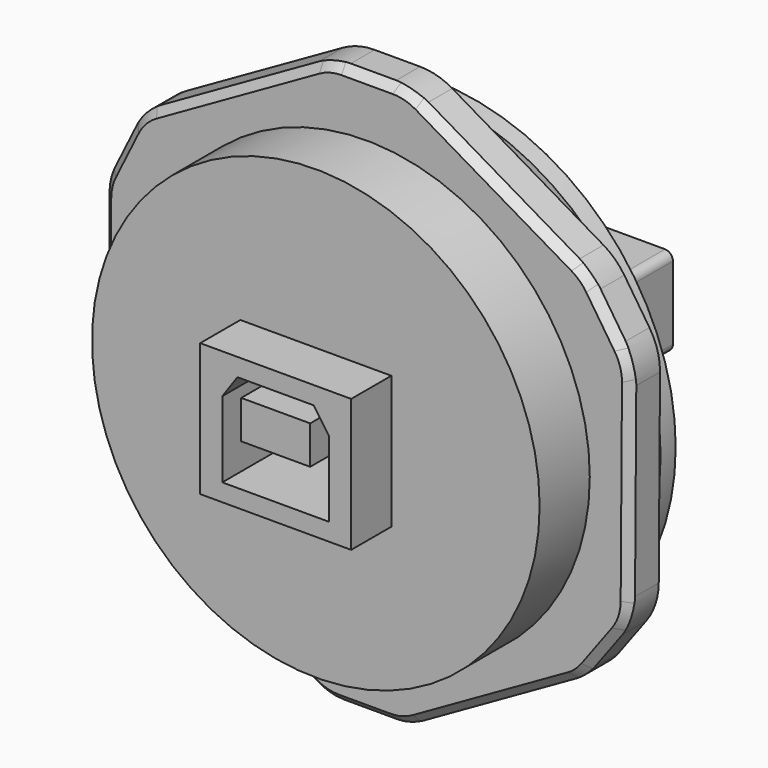
from build123d import *

# Parameters (mm, degrees)
F0_R      = 17.85
F1_DEPTH  = 5
F4_DEPTH  = 3
F5_SIZE   = 0.635
F6_F1_R   = 5.08
F6_F2_R   = 5.08
F6_F3_R   = 5.08
F6_F4_R   = 5.08
F6_F5_R   = 5.08
F6_F6_R   = 5.08
F6_F7_R   = 5.08
F6_F8_R   = 5.08
F6_F9_R   = 5.08
F6_F10_R  = 5.08
F6_F11_R  = 5.08
F6_F12_R  = 5.08
F6_F13_R  = 5.08
F6_F14_R  = 5.08
F6_F15_R  = 5.08
F6_F16_R  = 5.08
F6_F17_R  = 5.08
F6_F18_R  = 5.08
F6_F19_R  = 5.08
F6_F20_R  = 5.08
F6_F21_R  = 5.08
F6_F22_R  = 5.08
F6_F23_R  = 5.08
F6_F24_R  = 5.08
F7_R      = 19.5
F8_DEPTH  = 1.5
F9_W      = 12.04
F9_H      = 10.6
F9_W_2    = 5.5
F9_H_2    = 3.05
F10_DEPTH = 4
F11_DEPTH = 3
F12_W     = 10
F12_H     = 1.5
F13_DEPTH = 15.1


with BuildPart() as f1:
    # F0 (on Front) → F1 (new body, symmetric)
    with BuildSketch(Plane.XZ):
        Circle(F0_R)
    extrude(amount=F1_DEPTH, both=True)

    # F3 (on offset) → F4 (join)
    with BuildSketch(Plane(origin=(0, 3, 0), x_dir=(-1, 0, 0), z_dir=(0, 1, 0))):
        Polygon((-3.2903481497, 22.4154013943), (-17.5555016387, 14.0492031865), (-21.0601798177, 8.7539476816), (-20.9370838593, -9.2984309735), (-17.1594677511, -14.4025583758), (-3.0596518503, -22.4154013943), (3.2903481497, -22.4154013943), (18.0473649217, -13.7607362086), (21.0561899697, -8.1688249226), (20.9448872454, 8.1540418144), (18.1346734923, 13.8483546493), (3.0596518503, 22.4154013943), align=None)
    extrude(amount=-F4_DEPTH)

    # F5
    f5_edges = [f1.edges().sort_by_distance(p)[0] for p in [
        (10.422925, 0, 18.232302),
        (19.307841, 0, 11.401575),
        (20.998632, 0, -0.272242),
        (19.048276, 0, -11.850495),
        (10.10956, 0, -18.40898),
        (-0.115348, 0, -22.415401),
        (-10.668857, 0, -18.088069),
        (-19.551777, 0, -10.964781),
        (-21.000539, 0, -0.007392),
        (-19.53978, 0, 11.001198),
        (-10.597163, 0, 18.131878),
        (0.115348, 0, 22.415401),
    ]]
    chamfer(f5_edges, length=F5_SIZE)

    # F6: fillet of radius 5.08 on 24 edges, made by hand

    # F6_f1
    f6_f1_edges = [f1.edges().sort_by_distance(p)[0] for p in [
        (-20.9448872454, 1.8175, 8.1540418144),
    ]]
    fillet(f6_f1_edges, radius=F6_F1_R)

    # F6_f2
    f6_f2_edges = [f1.edges().sort_by_distance(p)[0] for p in [
        (-18.1346734923, 1.8175, 13.8483546493),
    ]]
    fillet(f6_f2_edges, radius=F6_F2_R)

    # F6_f3
    f6_f3_edges = [f1.edges().sort_by_distance(p)[0] for p in [
        (-21.0561899697, 1.8175, -8.1688249226),
    ]]
    fillet(f6_f3_edges, radius=F6_F3_R)

    # F6_f4
    f6_f4_edges = [f1.edges().sort_by_distance(p)[0] for p in [
        (-20.5635101748, 0.2530156874, 8.0636856851),
    ]]
    fillet(f6_f4_edges, radius=F6_F4_R)

    # F6_f5
    f6_f5_edges = [f1.edges().sort_by_distance(p)[0] for p in [
        (-17.80801976, 0.205710524, 13.540221636),
    ]]
    fillet(f6_f5_edges, radius=F6_F5_R)

    # F6_f6
    f6_f6_edges = [f1.edges().sort_by_distance(p)[0] for p in [
        (-3.0596518503, 1.8175, 22.4154013943),
    ]]
    fillet(f6_f6_edges, radius=F6_F6_R)

    # F6_f7
    f6_f7_edges = [f1.edges().sort_by_distance(p)[0] for p in [
        (-18.0473649217, 1.8175, -13.7607362086),
    ]]
    fillet(f6_f7_edges, radius=F6_F7_R)

    # F6_f8
    f6_f8_edges = [f1.edges().sort_by_distance(p)[0] for p in [
        (-20.6589027008, 0.2383946915, -8.0701656315),
    ]]
    fillet(f6_f8_edges, radius=F6_F8_R)

    # F6_f9
    f6_f9_edges = [f1.edges().sort_by_distance(p)[0] for p in [
        (-2.9534511203, 0.2331786487, 22.013580043),
    ]]
    fillet(f6_f9_edges, radius=F6_F9_R)

    # F6_f10
    f6_f10_edges = [f1.edges().sort_by_distance(p)[0] for p in [
        (3.2903481497, 1.8175, 22.4154013943),
    ]]
    fillet(f6_f10_edges, radius=F6_F10_R)

    # F6_f11
    f6_f11_edges = [f1.edges().sort_by_distance(p)[0] for p in [
        (-3.2903481497, 1.8175, -22.4154013943),
    ]]
    fillet(f6_f11_edges, radius=F6_F11_R)

    # F6_f12
    f6_f12_edges = [f1.edges().sort_by_distance(p)[0] for p in [
        (17.5555016387, 1.8175, 14.0492031865),
    ]]
    fillet(f6_f12_edges, radius=F6_F12_R)

    # F6_f13
    f6_f13_edges = [f1.edges().sort_by_distance(p)[0] for p in [
        (3.0596518503, 1.8175, -22.4154013943),
    ]]
    fillet(f6_f13_edges, radius=F6_F13_R)

    # F6_f14
    f6_f14_edges = [f1.edges().sort_by_distance(p)[0] for p in [
        (21.0601798177, 1.8175, 8.7539476816),
    ]]
    fillet(f6_f14_edges, radius=F6_F14_R)

    # F6_f15
    f6_f15_edges = [f1.edges().sort_by_distance(p)[0] for p in [
        (17.1594677511, 1.8175, -14.4025583758),
    ]]
    fillet(f6_f15_edges, radius=F6_F15_R)

    # F6_f16
    f6_f16_edges = [f1.edges().sort_by_distance(p)[0] for p in [
        (20.9370838593, 1.8175, -9.2984309735),
    ]]
    fillet(f6_f16_edges, radius=F6_F16_R)

    # F6_f17
    f6_f17_edges = [f1.edges().sort_by_distance(p)[0] for p in [
        (-17.7394232188, 0.2231799565, -13.4639178232),
    ]]
    fillet(f6_f17_edges, radius=F6_F17_R)

    # F6_f18
    f6_f18_edges = [f1.edges().sort_by_distance(p)[0] for p in [
        (3.1799932747, 0.2286960306, 22.009097425),
    ]]
    fillet(f6_f18_edges, radius=F6_F18_R)

    # F6_f19
    f6_f19_edges = [f1.edges().sort_by_distance(p)[0] for p in [
        (17.2850276, 0.2518471741, 13.7636444987),
    ]]
    fillet(f6_f19_edges, radius=F6_F19_R)

    # F6_f20
    f6_f20_edges = [f1.edges().sort_by_distance(p)[0] for p in [
        (20.6315309968, 0.2072299177, 8.6265365553),
    ]]
    fillet(f6_f20_edges, radius=F6_F20_R)

    # F6_f21
    f6_f21_edges = [f1.edges().sort_by_distance(p)[0] for p in [
        (20.4954738766, 0.1923957856, -9.1511150124),
    ]]
    fillet(f6_f21_edges, radius=F6_F21_R)

    # F6_f22
    f6_f22_edges = [f1.edges().sort_by_distance(p)[0] for p in [
        (16.9069384559, 0.262522864, -14.1176463871),
    ]]
    fillet(f6_f22_edges, radius=F6_F22_R)

    # F6_f23
    f6_f23_edges = [f1.edges().sort_by_distance(p)[0] for p in [
        (2.9534511203, 0.2331786487, -22.013580043),
    ]]
    fillet(f6_f23_edges, radius=F6_F23_R)

    # F6_f24
    f6_f24_edges = [f1.edges().sort_by_distance(p)[0] for p in [
        (-3.1799932747, 0.2286960306, -22.009097425),
    ]]
    fillet(f6_f24_edges, radius=F6_F24_R)

    # F7 (on face) → F8 (join)
    with BuildSketch(Plane(origin=(0, 5, 0), x_dir=(-1, 0, 0), z_dir=(0, 1, 0))):
        Circle(F7_R)
    extrude(amount=F8_DEPTH)

    # F9 (on face) → F10 (join)
    with BuildSketch(Plane.XZ.offset(5)):
        Rectangle(F9_W, F9_H)
        Polygon((4.2387, -3.903), (-4.2613, -3.903), (-4.2613, 2.1469455678), (-3.0499028451, 3.877), (3.0273028451, 3.877), (4.2387, 2.1469455678), align=None, mode=Mode.SUBTRACT)
        with Locations((0, 0.9936958086)):
            Rectangle(F9_W_2, F9_H_2)
    extrude(amount=F10_DEPTH)

    # F9 (on face) → F11 (cut)
    with BuildSketch(Plane.XZ.offset(5)):
        Polygon((-4.2613, 2.1469455678), (-4.2613, -3.903), (4.2387, -3.903), (4.2387, 2.1469455678), (3.0273028451, 3.877), (-3.0499028451, 3.877), align=None)
        with Locations((0, 0.9936958086)):
            Rectangle(F9_W_2, F9_H_2, mode=Mode.SUBTRACT)
    extrude(amount=-F11_DEPTH, mode=Mode.SUBTRACT)

    # F12 (on face) → F13 (join)
    with BuildSketch(Plane(origin=(0, 6.5, 0), x_dir=(-1, 0, 0), z_dir=(0, 1, 0))):
        with BuildLine():
            Line((6.565, 3.55), (-6.565, 3.55))
            ThreePointArc((-6.565, 3.55), (-7.0140128061, 3.3640128061), (-7.2, 2.915))
            Line((-7.2, 2.915), (-7.2, -2.915))
            ThreePointArc((-7.2, -2.915), (-7.0140128061, -3.3640128061), (-6.565, -3.55))
            Line((-6.565, -3.55), (6.565, -3.55))
            ThreePointArc((6.565, -3.55), (7.0140128061, -3.3640128061), (7.2, -2.915))
            Line((7.2, -2.915), (7.2, 2.915))
            ThreePointArc((7.2, 2.915), (7.0140128061, 3.3640128061), (6.565, 3.55))
        make_face()
        with BuildLine():
            ThreePointArc((-6.95, 2.665), (-6.7640128061, 3.1140128061), (-6.315, 3.3))
            Line((-6.315, 3.3), (6.315, 3.3))
            ThreePointArc((6.315, 3.3), (6.7640128061, 3.1140128061), (6.95, 2.665))
            Line((6.95, 2.665), (6.95, -2.665))
            ThreePointArc((6.95, -2.665), (6.7640128061, -3.1140128061), (6.315, -3.3))
            Line((6.315, -3.3), (-6.315, -3.3))
            ThreePointArc((-6.315, -3.3), (-6.7640128061, -3.1140128061), (-6.95, -2.665))
            Line((-6.95, -2.665), (-6.95, 2.665))
        make_face(mode=Mode.SUBTRACT)
        with Locations((0, 0.7)):
            Rectangle(F12_W, F12_H)
    extrude(amount=F13_DEPTH)


solid = f1.part
